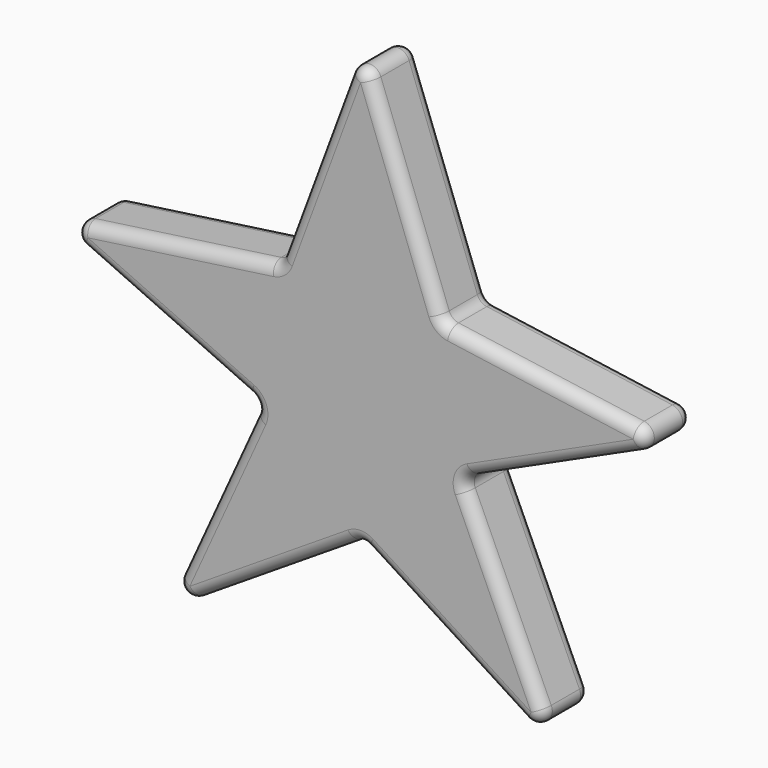
from build123d import *

# Parameters (mm, degrees)
F1_DEPTH = 6.35
F2_R     = 1.27


with BuildPart() as f1:
    # F0 (on Front) → F1 (new body)
    with BuildSketch(Plane.XZ):
        Polygon((0, 28.9144045194), (-8.8481841409, 5.1053802343), (-33.9983782601, 1.5518276782), (-10.8810784623, -8.9719762946), (-21.404882435, -32.0892760924), (0, -18.4148105473), align=None)
        Polygon((8.8481841409, 5.1053802343), (0, 28.9144045194), (0, -18.4148105473), (21.404882435, -32.0892760924), (10.8810784623, -8.9719762946), (33.9983782601, 1.5518276782), align=None)
    extrude(amount=F1_DEPTH)

    # F2
    f2_edges = [f1.edges().sort_by_distance(p)[0] for p in [
        (-10.702441, 0, -25.252043),
        (-10.702441, -6.35, -25.252043),
        (10.702441, 0, -25.252043),
        (10.702441, -6.35, -25.252043),
        (16.14298, 0, -20.530626),
        (16.14298, -6.35, -20.530626),
        (22.439728, -6.35, -3.710074),
        (22.439728, 0, -3.710074),
        (21.423281, -6.35, 3.328604),
        (21.423281, 0, 3.328604),
        (0, -3.175, 28.914405),
        (-8.848184, -3.175, 5.10538),
        (-4.424092, 0, 17.009892),
        (-4.424092, -6.35, 17.009892),
        (8.848184, -3.175, 5.10538),
        (4.424092, 0, 17.009892),
        (4.424092, -6.35, 17.009892),
        (10.881078, -3.175, -8.971976),
        (33.998378, -3.175, 1.551828),
        (21.404882, -3.175, -32.089276),
        (0, -3.175, -18.414811),
        (-10.881078, -3.175, -8.971976),
        (-21.404882, -3.175, -32.089276),
        (-16.14298, 0, -20.530626),
        (-16.14298, -6.35, -20.530626),
        (-33.998378, -3.175, 1.551828),
        (-21.423281, 0, 3.328604),
        (-21.423281, -6.35, 3.328604),
        (-22.439728, 0, -3.710074),
        (-22.439728, -6.35, -3.710074),
    ]]
    fillet(f2_edges, radius=F2_R)


solid = f1.part
